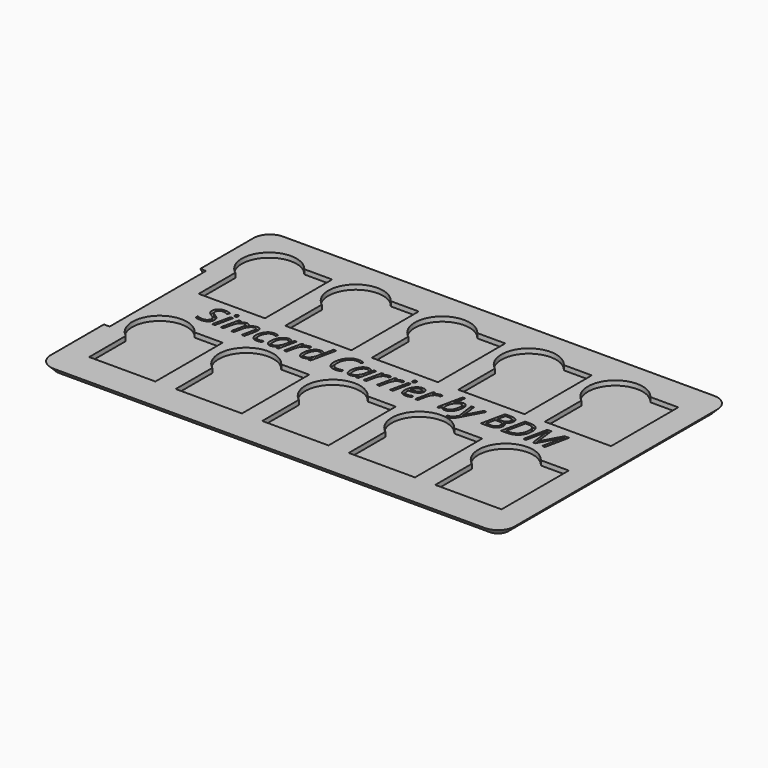
from build123d import *

# Parameters (mm, degrees)
F1_DEPTH     = 0.3
F3_DEPTH     = 0.85
F4_SIZE      = 1.14999
F5_W         = 1.05
F5_H         = 22
F6_DEPTH     = 25
F7_TEXT_SIZE = 6.1108006371
F8_DEPTH     = 0.5


# Not quite as in the source:
# - a fillet or chamfer is up to 0.001 mm smaller than in the source, because OpenCascade refuses the exact size
# - a feature names something its author has since deleted; it is built from what else it names
# - Text() gives the source's letters only with a copy of the font that has no kerning and outlines rounded to 1/6400 em; it was checked with that copy


with BuildPart() as f1:
    # F0 (on Top) → F1 (new body)
    with BuildSketch(Plane.XY):
        with BuildLine():
            ThreePointArc((0, 3), (0.8786796564, 0.8786796564), (3, 0))
            Line((3, 0), (81.7, 0))
            ThreePointArc((81.7, 0), (83.8213203436, 0.8786796564), (84.7, 3))
            Line((84.7, 3), (84.7, 49.3))
            ThreePointArc((84.7, 49.3), (83.8213203436, 51.4213203436), (81.7, 52.3))
            Line((81.7, 52.3), (3, 52.3))
            ThreePointArc((3, 52.3), (0.8786796564, 51.4213203436), (0, 49.3))
            Line((0, 49.3), (0, 3))
        make_face()
    extrude(amount=F1_DEPTH)

    # F2 (on face) → F3 (join)
    with BuildSketch(Plane.XY.offset(0.3)):
        with BuildLine():
            Line((0, 49.3), (0, 3))
            ThreePointArc((0, 3), (0.8786796564, 0.8786796564), (3, 0))
            Line((3, 0), (81.7, 0))
            ThreePointArc((81.7, 0), (83.8213203436, 0.8786796564), (84.7, 3))
            Line((84.7, 3), (84.7, 49.3))
            ThreePointArc((84.7, 49.3), (83.8213203436, 51.4213203436), (81.7, 52.3))
            Line((81.7, 52.3), (3, 52.3))
            ThreePointArc((3, 52.3), (0.8786796564, 51.4213203436), (0, 49.3))
        make_face()
        with BuildLine():
            Line((11.6499995515, 21.325), (16.7499995515, 21.325))
            Line((16.7499995515, 21.325), (16.7499995515, 5.975))
            Line((16.7499995515, 5.975), (4.6499995515, 5.975))
            Line((4.6499995515, 5.975), (4.6499995515, 14.325))
            ThreePointArc((4.6499995515, 14.325), (4.1144656455, 21.8605339059), (11.6499995515, 21.325))
        make_face(mode=Mode.SUBTRACT)
        with BuildLine():
            Line((27.4499995515, 21.325), (32.5499995515, 21.325))
            Line((32.5499995515, 21.325), (32.5499995515, 5.975))
            Line((32.5499995515, 5.975), (20.4499995515, 5.975))
            Line((20.4499995515, 5.975), (20.4499995515, 14.325))
            ThreePointArc((20.4499995515, 14.325), (19.9144656455, 21.8605339059), (27.4499995515, 21.325))
        make_face(mode=Mode.SUBTRACT)
        with BuildLine():
            Line((43.2499995515, 21.325), (48.3499995515, 21.325))
            Line((48.3499995515, 21.325), (48.3499995515, 5.975))
            Line((48.3499995515, 5.975), (36.2499995515, 5.975))
            Line((36.2499995515, 5.975), (36.2499995515, 14.325))
            ThreePointArc((36.2499995515, 14.325), (35.7144656455, 21.8605339059), (43.2499995515, 21.325))
        make_face(mode=Mode.SUBTRACT)
        with BuildLine():
            Line((59.0499995515, 21.325), (64.1499995515, 21.325))
            Line((64.1499995515, 21.325), (64.1499995515, 5.975))
            Line((64.1499995515, 5.975), (52.0499995515, 5.975))
            Line((52.0499995515, 5.975), (52.0499995515, 14.325))
            ThreePointArc((52.0499995515, 14.325), (51.5144656455, 21.8605339059), (59.0499995515, 21.325))
        make_face(mode=Mode.SUBTRACT)
        with BuildLine():
            Line((74.8499995515, 21.325), (79.9499995515, 21.325))
            Line((79.9499995515, 21.325), (79.9499995515, 5.975))
            Line((79.9499995515, 5.975), (67.8499995515, 5.975))
            Line((67.8499995515, 5.975), (67.8499995515, 14.325))
            ThreePointArc((67.8499995515, 14.325), (67.3144656455, 21.8605339059), (74.8499995515, 21.325))
        make_face(mode=Mode.SUBTRACT)
        with BuildLine():
            Line((11.6499995515, 46.325), (16.7499995515, 46.325))
            Line((16.7499995515, 46.325), (16.7499995515, 30.975))
            Line((16.7499995515, 30.975), (4.6499995515, 30.975))
            Line((4.6499995515, 30.975), (4.6499995515, 39.325))
            ThreePointArc((4.6499995515, 39.325), (4.1144656455, 46.8605339059), (11.6499995515, 46.325))
        make_face(mode=Mode.SUBTRACT)
        with BuildLine():
            Line((27.4499995515, 46.325), (32.5499995515, 46.325))
            Line((32.5499995515, 46.325), (32.5499995515, 30.975))
            Line((32.5499995515, 30.975), (20.4499995515, 30.975))
            Line((20.4499995515, 30.975), (20.4499995515, 39.325))
            ThreePointArc((20.4499995515, 39.325), (19.9144656455, 46.8605339059), (27.4499995515, 46.325))
        make_face(mode=Mode.SUBTRACT)
        with BuildLine():
            Line((43.2499995515, 46.325), (48.3499995515, 46.325))
            Line((48.3499995515, 46.325), (48.3499995515, 30.975))
            Line((48.3499995515, 30.975), (36.2499995515, 30.975))
            Line((36.2499995515, 30.975), (36.2499995515, 39.325))
            ThreePointArc((36.2499995515, 39.325), (35.7144656455, 46.8605339059), (43.2499995515, 46.325))
        make_face(mode=Mode.SUBTRACT)
        with BuildLine():
            Line((59.0499995515, 46.325), (64.1499995515, 46.325))
            Line((64.1499995515, 46.325), (64.1499995515, 30.975))
            Line((64.1499995515, 30.975), (52.0499995515, 30.975))
            Line((52.0499995515, 30.975), (52.0499995515, 39.325))
            ThreePointArc((52.0499995515, 39.325), (51.5144656455, 46.8605339059), (59.0499995515, 46.325))
        make_face(mode=Mode.SUBTRACT)
        with BuildLine():
            Line((74.8499995515, 46.325), (79.9499995515, 46.325))
            Line((79.9499995515, 46.325), (79.9499995515, 30.975))
            Line((79.9499995515, 30.975), (67.8499995515, 30.975))
            Line((67.8499995515, 30.975), (67.8499995515, 39.325))
            ThreePointArc((67.8499995515, 39.325), (67.3144656455, 46.8605339059), (74.8499995515, 46.325))
        make_face(mode=Mode.SUBTRACT)
    extrude(amount=F3_DEPTH)

    # F4 (size 1.15 in the source; OpenCascade refuses exactly that, so slightly less here)
    f4_edges = [f1.edges().sort_by_distance(p)[0] for p in [
        (42.35, 0, 0),
    ]]
    chamfer(f4_edges, length=F4_SIZE)

    # F5 (on face) → F6 (cut)
    with BuildSketch(Plane.XY.offset(1.15)):
        with Locations((0.525, 26.15)):
            Rectangle(F5_W, F5_H)
    extrude(amount=-F6_DEPTH, mode=Mode.SUBTRACT)

    # F7 (on face) → F8 (cut)
    with BuildSketch(Plane.XY.offset(1.15)):
        with Locations((8.7466267869, 24.8791929334)):
            Text('Simcard Carrier by BDM', F7_TEXT_SIZE, font='Open Sans', font_style=FontStyle.ITALIC, text_align=(TextAlign.LEFT, TextAlign.BOTTOM))
    extrude(amount=-F8_DEPTH, mode=Mode.SUBTRACT)


solid = f1.part
